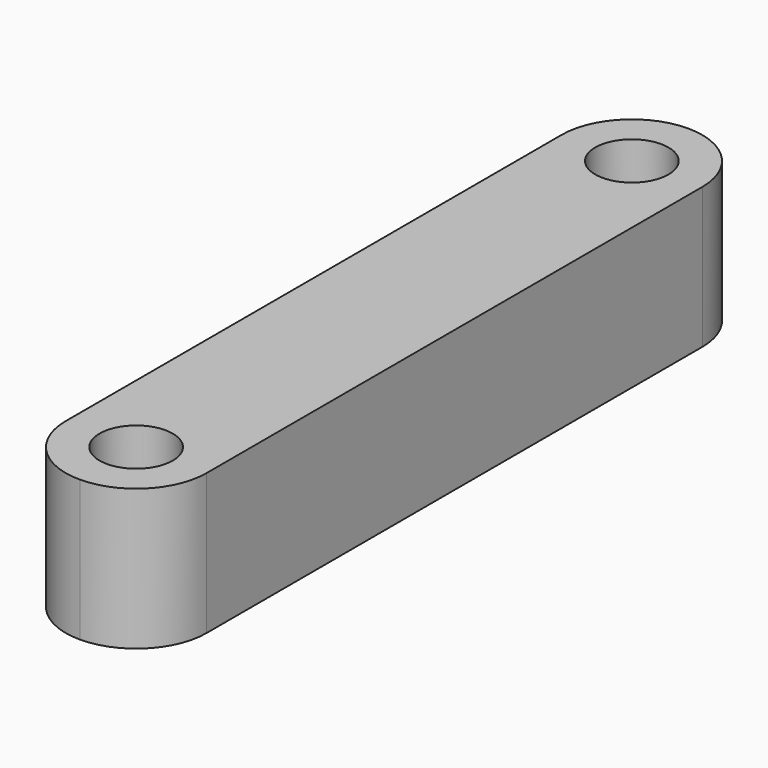
from build123d import *

# Parameters (mm, degrees)
F0_W     = 6.35
F0_H     = 34.29
F1_DEPTH = 6.35
F2_R     = 3.17499
F3_R     = 1.651
F4_DEPTH = 6.35


# Not quite as in the source:
# - a fillet or chamfer is up to 0.001 mm smaller than in the source, because OpenCascade refuses the exact size


with BuildPart() as f1:
    # F0 (on Top) → F1 (new body)
    with BuildSketch(Plane.XY):
        Rectangle(F0_W, F0_H)
    extrude(amount=F1_DEPTH)

    # F2 (radius 3.175 in the source; OpenCascade refuses exactly that, so slightly less here)
    f2_edges = [f1.edges().sort_by_distance(p)[0] for p in [
        (3.175, 17.145, 3.175),
        (-3.175, 17.145, 3.175),
        (3.175, -17.145, 3.175),
        (-3.175, -17.145, 3.175),
    ]]
    fillet(f2_edges, radius=F2_R)

    # F3 (on face) → F4 (cut, through all)
    with BuildSketch(Plane.XY.offset(6.35)):
        with Locations((0, -13.97)):
            Circle(F3_R)
        with Locations((0, 13.97)):
            Circle(F3_R)
    extrude(amount=-F4_DEPTH, mode=Mode.SUBTRACT)


solid = f1.part
